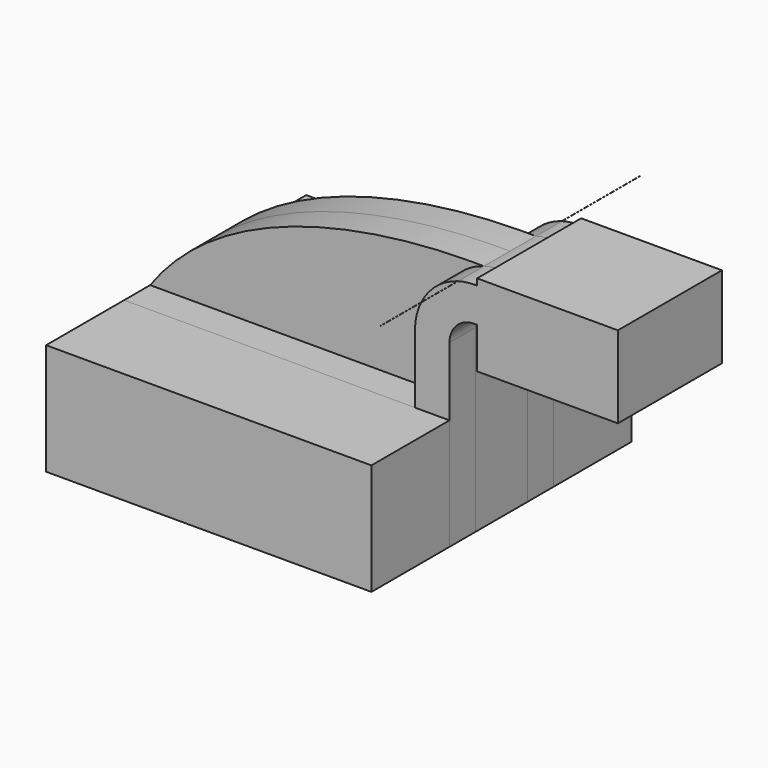
from build123d import *

# Parameters (mm, degrees)
F1_DEPTH = 63.5
F2_DEPTH = 25.4
F3_DEPTH = 12.7


with BuildPart() as f1:
    # F0 (on Front) → F1 (new body, symmetric)
    with BuildSketch(Plane.XZ):
        Polygon((-63.5346770287, 21.7547100037), (-63.5346770287, -21.7547100037), (63.5346770287, -21.7547100037), (63.5346770287, 21.7547100037), (50.0744320452, 21.7547100037), align=None)
    extrude(amount=F1_DEPTH, both=True)


with BuildPart() as f1b:
    # F0 (on Front) → F1, piece 2 (new body, symmetric)
    with BuildSketch(Plane.XZ):
        with BuildLine():
            ThreePointArc((66.8844246133, 70.6885641711), (66.835957909, 70.6747977575), (66.7875213509, 70.6609256486))
            add(Edge.make_bspline(
                [(66.7875213509, 70.6609256486), (66.8542987198, 70.666627221), (66.8577943875, 70.675737456), (66.8844246133, 70.6885641711)],
                knots=[0.9737991277, 0.9737991277, 0.9737991277, 0.9737991277, 1, 1, 1, 1], degree=3))
        make_face()
    extrude(amount=F1_DEPTH, both=True)


with BuildPart() as f2:
    # F0 (on Front) → F2 (new body, symmetric)
    with BuildSketch(Plane.XZ):
        with BuildLine():
            ThreePointArc((66.8844246133, 70.6885641711), (66.835957909, 70.6747977575), (66.7875213509, 70.6609256486))
            add(Edge.make_bspline(
                [(66.7875213509, 70.6609256486), (66.8542987198, 70.666627221), (66.8577943875, 70.675737456), (66.8844246133, 70.6885641711)],
                knots=[0.9737991277, 0.9737991277, 0.9737991277, 0.9737991277, 1, 1, 1, 1], degree=3))
        make_face()
        Polygon((-63.5346770287, 21.7547100037), (-63.5346770287, -21.7547100037), (63.5346770287, -21.7547100037), (63.5346770287, 21.7547100037), (50.0744320452, 21.7547100037), align=None)
        with BuildLine():
            Line((50.0744320452, 21.7547100037), (63.5346770287, 21.7547100037))
            Line((63.5346770287, 21.7547100037), (63.5346770287, 48.4641493763))
            ThreePointArc((63.5346770287, 48.4641493763), (66.3570400807, 55.2779365345), (73.1708272389, 58.1002995865))
            Line((73.1708272389, 58.1002995865), (74.3306106452, 58.1002995865))
            Line((74.3306106452, 58.1002995865), (74.3306106452, 71.5605445699))
            Line((74.3306106452, 71.5605445699), (73.1708272389, 71.5605445699))
            ThreePointArc((73.1708272389, 71.5605445699), (69.9975321145, 71.3415108718), (66.8844246133, 70.6885641711))
            add(Edge.make_bspline(
                [(66.7875213509, 70.6609256486), (66.8542987198, 70.666627221), (66.8577943875, 70.675737456), (66.8844246133, 70.6885641711)],
                knots=[0.9737991277, 0.9737991277, 0.9737991277, 0.9737991277, 1, 1, 1, 1], degree=3))
            ThreePointArc((66.7875213509, 70.6609256486), (54.7198811063, 62.3568113874), (50.0744320452, 48.4641493763))
            Line((50.0744320452, 48.4641493763), (50.0744320452, 21.7547100037))
        make_face()
        Polygon((74.3306106452, 71.5605445699), (74.3306106452, 58.1002995865), (74.3306106452, 42.1084646629), (129.3090334657, 42.1084646629), (129.3090334657, 74.0921345101), (74.3306106452, 74.0921345101), align=None)
    extrude(amount=F2_DEPTH, both=True)


with BuildPart() as f3:
    # F0 (on Front) → F3 (new body, symmetric)
    with BuildSketch(Plane.XZ):
        with BuildLine():
            ThreePointArc((66.8844246133, 70.6885641711), (66.835957909, 70.6747977575), (66.7875213509, 70.6609256486))
            add(Edge.make_bspline(
                [(66.7875213509, 70.6609256486), (66.8542987198, 70.666627221), (66.8577943875, 70.675737456), (66.8844246133, 70.6885641711)],
                knots=[0.9737991277, 0.9737991277, 0.9737991277, 0.9737991277, 1, 1, 1, 1], degree=3))
        make_face()
        Polygon((-63.5346770287, 21.7547100037), (-63.5346770287, -21.7547100037), (63.5346770287, -21.7547100037), (63.5346770287, 21.7547100037), (50.0744320452, 21.7547100037), align=None)
        with BuildLine():
            Line((50.0744320452, 21.7547100037), (63.5346770287, 21.7547100037))
            Line((63.5346770287, 21.7547100037), (63.5346770287, 48.4641493763))
            ThreePointArc((63.5346770287, 48.4641493763), (66.3570400807, 55.2779365345), (73.1708272389, 58.1002995865))
            Line((73.1708272389, 58.1002995865), (74.3306106452, 58.1002995865))
            Line((74.3306106452, 58.1002995865), (74.3306106452, 71.5605445699))
            Line((74.3306106452, 71.5605445699), (73.1708272389, 71.5605445699))
            ThreePointArc((73.1708272389, 71.5605445699), (69.9975321145, 71.3415108718), (66.8844246133, 70.6885641711))
            add(Edge.make_bspline(
                [(66.7875213509, 70.6609256486), (66.8542987198, 70.666627221), (66.8577943875, 70.675737456), (66.8844246133, 70.6885641711)],
                knots=[0.9737991277, 0.9737991277, 0.9737991277, 0.9737991277, 1, 1, 1, 1], degree=3))
            ThreePointArc((66.7875213509, 70.6609256486), (54.7198811063, 62.3568113874), (50.0744320452, 48.4641493763))
            Line((50.0744320452, 48.4641493763), (50.0744320452, 21.7547100037))
        make_face()
        with BuildLine():
            add(Edge.make_bspline(
                [(-63.5346770287, 21.7547100037), (-25.5911517888, 74.9457031488), (64.3056290338, 70.4490171987), (66.7875213509, 70.6609256486)],
                knots=[0, 0, 0, 0, 0.9737991277, 0.9737991277, 0.9737991277, 0.9737991277], degree=3))
            Line((-63.5346770287, 21.7547100037), (50.0744320452, 21.7547100037))
            Line((50.0744320452, 21.7547100037), (50.0744320452, 48.4641493763))
            ThreePointArc((50.0744320452, 48.4641493763), (54.7198811063, 62.3568113874), (66.7875213509, 70.6609256486))
        make_face()
    extrude(amount=F3_DEPTH, both=True)


solid = Compound([f1.part, f1b.part, f2.part, f3.part])
